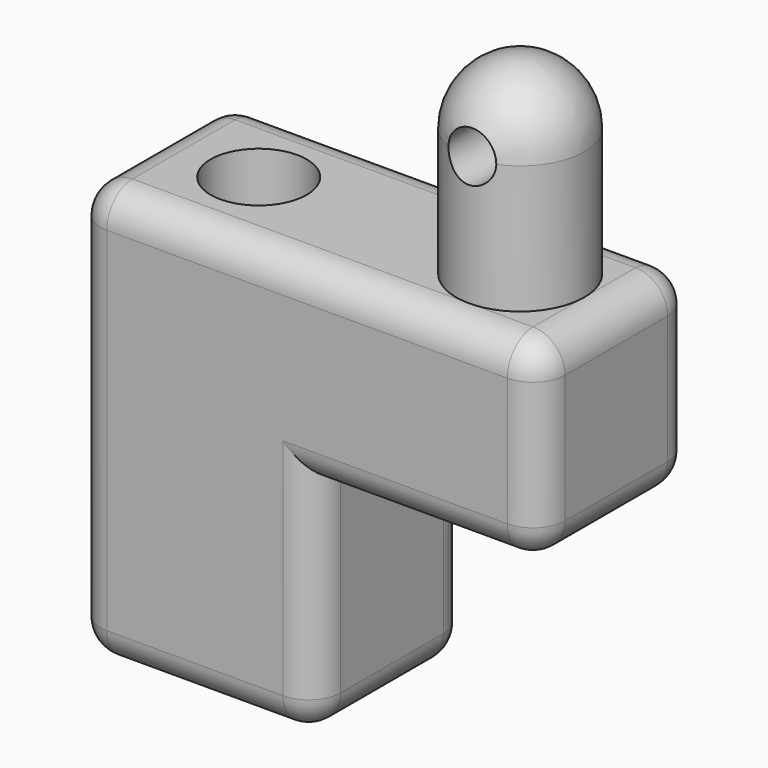
from build123d import *

# Parameters (mm, degrees)
F1_DEPTH = 3
F2_R     = 2
F3_DEPTH = 6
F4_R     = 2
F6_DEPTH = 12.5
F8_D     = 3
F9_R     = 0.99999


# Not quite as in the source:
# - a fillet or chamfer is up to 0.001 mm smaller than in the source, because OpenCascade refuses the exact size


with BuildPart() as f1:
    # F0 (on Front) → F1 (new body, symmetric)
    with BuildSketch(Plane.XZ):
        Polygon((0, 13), (0, 0), (7.5, 0), (7.5, 7), (14.5, 7), (14.5, 13), align=None)
    extrude(amount=F1_DEPTH, both=True)

    # F2 (on face) → F3 (join)
    with BuildSketch(Plane.XY.offset(13)):
        with Locations((11.5, 0)):
            Circle(F2_R)
    extrude(amount=F3_DEPTH)

    # F4
    f4_edges = [f1.edges().sort_by_distance(p)[0] for p in [
        (9.5, 0, 19),
    ]]
    fillet(f4_edges, radius=F4_R)

    # F5 (on Front) → F6 (cut, symmetric)
    with BuildSketch(Plane.XZ):
        with BuildLine():
            Line((10.7404427901, 17), (12.2404427901, 17))
            ThreePointArc((12.2404427901, 17), (11.4904427901, 17.75), (10.7404427901, 17))
        make_face()
        with BuildLine():
            ThreePointArc((10.7404427901, 17), (11.4904427901, 16.25), (12.2404427901, 17))
            Line((12.2404427901, 17), (10.7404427901, 17))
        make_face()
    extrude(amount=F6_DEPTH, both=True, mode=Mode.SUBTRACT)

    # F8 (through all)
    with Locations(Plane(origin=(0, 0, 0), x_dir=(1, 0, 0), z_dir=(0, 0, -1))):
        with Locations((3.3399870154, 0)):
            Hole(F8_D / 2)

    # F9 (radius 1 in the source; OpenCascade refuses exactly that, so slightly less here)
    f9_edges = [f1.edges().sort_by_distance(p)[0] for p in [
        (0, 3, 6.5),
        (7.25, 3, 13),
        (14.5, 3, 10),
        (11, 3, 7),
        (3.75, 3, 0),
        (7.5, 3, 3.5),
        (0, -3, 6.5),
        (7.5, -3, 3.5),
        (3.75, -3, 0),
        (7.25, -3, 13),
        (14.5, -3, 10),
        (0, 0, 13),
        (0, 0, 0),
        (7.5, 0, 0),
        (11, -3, 7),
        (14.5, 0, 13),
        (14.5, 0, 7),
    ]]
    fillet(f9_edges, radius=F9_R)


solid = f1.part
